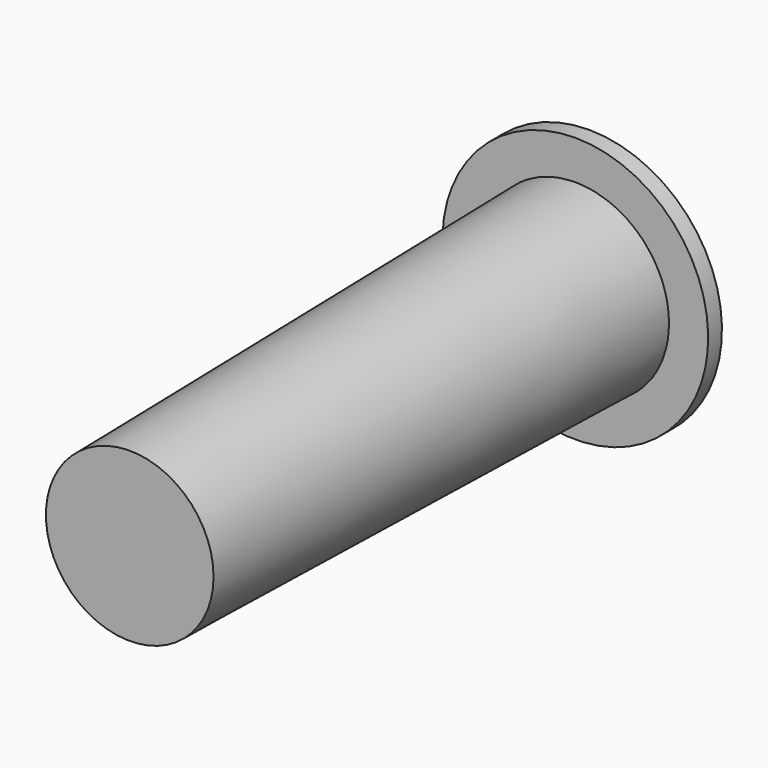
from build123d import *

# Parameters (mm, degrees)
F0_R     = 3.75
F2_R     = 3.25
F4_W     = 0.8722444763
F4_H     = 2.8718363028
F6_T     = 1
F7_W     = 1.1980372947
F7_H     = 13.454537373
F8_DEPTH = 12.5


with BuildPart() as f3:
    # F0 (on Front) → F3 section 0
    with BuildSketch(Plane.XZ):
        Circle(F0_R)
    # F2 (on offset) → F3 section 1
    with BuildSketch(Plane.XZ.offset(28)):
        Circle(F2_R)
    loft()

    # F6 (hollow, outwards: the wall grows on the outside; the body as it was is the cavity)
    f6_inside = f3.part
    offset(amount=F6_T, kind=Kind.INTERSECTION)
    add(f6_inside, mode=Mode.SUBTRACT)

    # F7 (on Right) → F8 (cut, symmetric)
    with BuildSketch(Plane.YZ):
        with Locations((0.5990186473, -5.23869e-05)):
            Rectangle(F7_W, F7_H)
    extrude(amount=F8_DEPTH, both=True, mode=Mode.SUBTRACT)


with BuildPart() as f5:
    # F4 (on Right) → F5 (revolve)
    with BuildSketch(Plane.YZ):
        with Locations((-0.4361222382, 5.2737850929)):
            Rectangle(F4_W, F4_H)
    revolve(axis=Axis((0, 0, 0), (0, -1, 0)))


solid = Compound([f3.part, f5.part])
